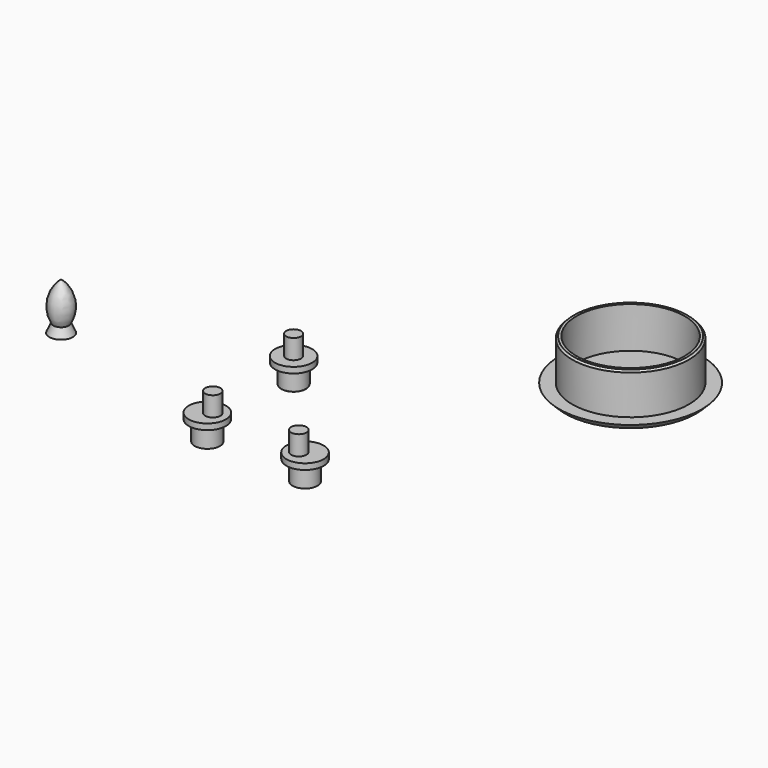
from build123d import *

# Parameters (mm, degrees)
F2_R      = 2
F3_DEPTH  = 15
F5_DEPTH  = 3.1
F6_R      = 6.45
F7_DEPTH  = 10
F9_R      = 0.5
F8_R      = 9.5
F10_DEPTH = 3
F11_R     = 3.8
F12_DEPTH = 10
F13_R     = 6.45
F14_DEPTH = 10
F15_R     = 9.5
F16_DEPTH = 3
F17_R     = 3.875
F18_DEPTH = 10
F19_R     = 6.35
F20_DEPTH = 10
F21_R     = 9.5
F22_DEPTH = 3
F23_R     = 3.89
F24_DEPTH = 10
F25_R     = 36.5
F26_DEPTH = 3
F27_R     = 29.85
F27_R_2   = 27.65
F28_DEPTH = 21
F29_SIZE  = 0.9
F30_SIZE  = 2.99999


# Not quite as in the source:
# - a fillet or chamfer is up to 0.001 mm smaller than in the source, because OpenCascade refuses the exact size


with BuildPart() as f1:
    # F0 (on Front) → F1 (revolve)
    with BuildSketch(Plane.XZ):
        with BuildLine():
            Line((6, 0), (3.9440578951, 4.5))
            ThreePointArc((3.9440578951, 4.5), (5.640035506, 14.9918887295), (0, 24))
            Line((0, 24), (0, 0))
            Line((0, 0), (6, 0))
        make_face()
    revolve(axis=Axis((0, 0, 12), (0, 0, 1)))

    # F2 (on face) → F3 (cut)
    with BuildSketch(Plane(origin=(0, 0, 0), x_dir=(1, 0, 0), z_dir=(0, 0, -1))):
        Circle(F2_R)
    extrude(amount=-F3_DEPTH, mode=Mode.SUBTRACT)

    # F4 (on face) → F5 (cut)
    with BuildSketch(Plane(origin=(0, 0, 15), x_dir=(1, 0, 0), z_dir=(0, 0, -1))):
        Polygon((3.55, 2.0495934556), (0, 4.0991869112), (-3.55, 2.0495934556), (-3.55, -2.0495934556), (0, -4.0991869112), (3.55, -2.0495934556), align=None)
    extrude(amount=F5_DEPTH, mode=Mode.SUBTRACT)


with BuildPart() as f7:
    # F6 (on Top) → F7 (new body)
    with BuildSketch(Plane.XY):
        with Locations((100.4927381873, 22.8593200445)):
            Circle(F6_R)
    extrude(amount=F7_DEPTH)

    # F9
    f9_edges = [f7.edges().sort_by_distance(p)[0] for p in [
        (94.042738, 22.85932, 0),
    ]]
    fillet(f9_edges, radius=F9_R)

    # F8 (on face) → F10 (join)
    with BuildSketch(Plane.XY.offset(10)):
        with Locations((100.4927381873, 22.8593200445)):
            Circle(F8_R)
    extrude(amount=F10_DEPTH)

    # F11 (on face) → F12 (join)
    with BuildSketch(Plane.XY.offset(13)):
        with Locations((100.4927381873, 22.8593200445)):
            Circle(F11_R)
    extrude(amount=F12_DEPTH)


with BuildPart() as f14:
    # F13 (on Top) → F14 (new body)
    with BuildSketch(Plane.XY):
        with Locations((104.1833385825, -36.8522368371)):
            Circle(F13_R)
    extrude(amount=F14_DEPTH)

    # F15 (on face) → F16 (join)
    with BuildSketch(Plane.XY.offset(10)):
        with Locations((104.1833385825, -36.8522368371)):
            Circle(F15_R)
    extrude(amount=F16_DEPTH)

    # F17 (on face) → F18 (join)
    with BuildSketch(Plane.XY.offset(13)):
        with Locations((106.1833385825, -35.8522368371)):
            Circle(F17_R)
    extrude(amount=F18_DEPTH)


with BuildPart() as f20:
    # F19 (on Top) → F20 (new body)
    with BuildSketch(Plane.XY):
        with Locations((156.1141461134, -39.3742509186)):
            Circle(F19_R)
    extrude(amount=F20_DEPTH)

    # F21 (on face) → F22 (join)
    with BuildSketch(Plane.XY.offset(10)):
        with Locations((156.1141461134, -39.3742509186)):
            Circle(F21_R)
    extrude(amount=F22_DEPTH)

    # F23 (on face) → F24 (join)
    with BuildSketch(Plane.XY.offset(13)):
        with Locations((153.9821015694, -40.6988210611)):
            Circle(F23_R)
    extrude(amount=F24_DEPTH)


with BuildPart() as f26:
    # F25 (on Top) → F26 (new body)
    with BuildSketch(Plane.XY):
        with Locations((207.9774290323, 103.7005186081)):
            Circle(F25_R)
    extrude(amount=F26_DEPTH)

    # F27 (on face) → F28 (join)
    with BuildSketch(Plane.XY.offset(3)):
        with Locations((207.9774290323, 103.7005186081)):
            Circle(F27_R)
        with Locations((207.9774290323, 103.7005186081)):
            Circle(F27_R_2, mode=Mode.SUBTRACT)
    extrude(amount=F28_DEPTH)

    # F29
    f29_edges = [f26.edges().sort_by_distance(p)[0] for p in [
        (178.127429, 103.700519, 24),
    ]]
    chamfer(f29_edges, length=F29_SIZE)

    # F30 (size 3 in the source; OpenCascade refuses exactly that, so slightly less here)
    f30_edges = [f26.edges().sort_by_distance(p)[0] for p in [
        (171.477429, 103.700519, 0),
    ]]
    chamfer(f30_edges, length=F30_SIZE)


solid = Compound([f1.part, f7.part, f14.part, f20.part, f26.part])
